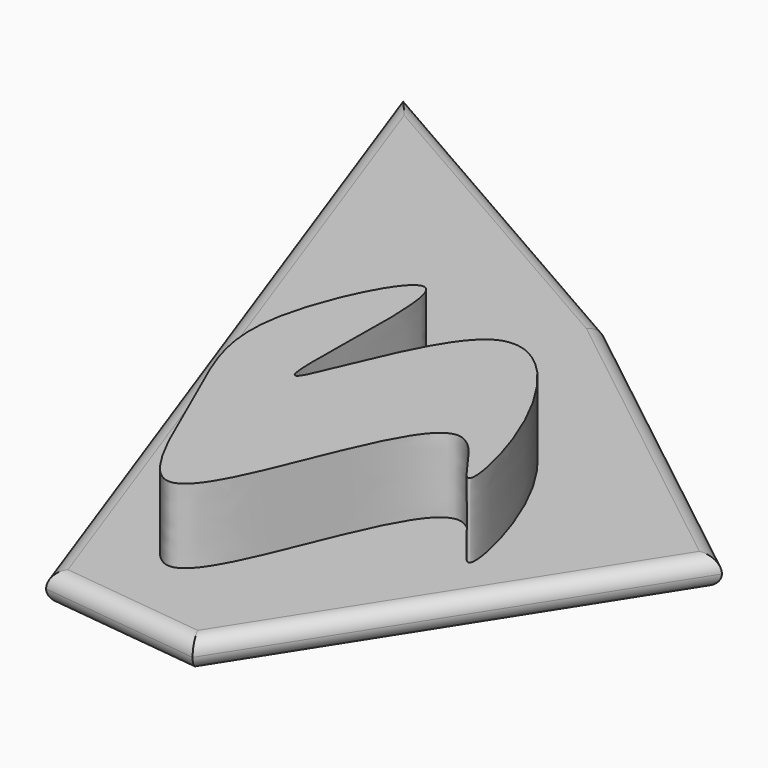
from build123d import *

# Parameters (mm, degrees)
F1_DEPTH    = 10
F2_R        = 5.08
F3_T1_DEPTH = 80.9842186748
F3_T3_DEPTH = 174.5076181059
F3_T5_DEPTH = 187.7665216843
F3_T7_DEPTH = 197.3953695309
F3_T9_DEPTH = 319.5650724593
F5_DEPTH    = 25.4


# Not quite as in the source:
# - a fillet or chamfer that OpenCascade refuses, or shapes differently, is made with other operations: its cross-section is extruded or revolved along the edge and cut away or added


with BuildPart() as f1:
    # F0 (on Top) → F1 (new body)
    with BuildSketch(Plane.XY):
        Polygon((96.3573604822, 27.2471159697), (-11.3680064678, 111.8755862117), (-138.5813802481, 184.7751736641), (-38.9760136604, -92.0266956091), (16.2400007248, -98.5227078199), align=None)
    extrude(amount=F1_DEPTH)

    # F2
    f2_edges = [f1.edges().sort_by_distance(p)[0] for p in [
        (-11.368006, -95.274702, 10),
        (56.298681, -35.637796, 10),
        (42.494677, 69.561351, 10),
        (-74.974693, 148.32538, 10),
        (-88.778697, 46.374239, 10),
    ]]
    fillet(f2_edges, radius=F2_R)

    # F3: fillet of radius 5.08 on 5 edges, made by hand

    # F3_s2 → F3_t1 (cut)
    with BuildSketch(Plane(origin=(-40.3717884669, 4.7496298633, 0), x_dir=(0, 0, 1), z_dir=(0.9931505824, -0.1168414342, 0))):
        with BuildLine():
            ThreePointArc((4.92, 95.9503796722), (1.4317675513, 94.4079813111), (0, 90.8728999824))
            Line((0, 90.8728999824), (-0.1016, 90.8728999824))
            Line((-0.1016, 90.8728999824), (-0.1016, 95.9503796722))
            Line((-0.1016, 95.9503796722), (0, 96.0519796722))
            ThreePointArc((0, 96.0519796722), (2.46, 96.0519796722), (4.9168, 96.051929266))
            Line((4.9168, 96.051929266), (4.92, 95.9503796722))
        make_face()
    extrude(amount=F3_T1_DEPTH, mode=Mode.SUBTRACT)

    # F3_s4 → F3_t3 (cut)
    with BuildSketch(Plane(origin=(-46.7764695351, -73.4306316227, 0), x_dir=(0, 0, 1), z_dir=(0.5372669108, 0.8434122755, 0))):
        with BuildLine():
            ThreePointArc((0, 61.5525271533), (1.4317675513, 65.0876084819), (4.92, 66.630006843))
            Line((4.92, 66.630006843), (4.9168, 66.7315564368))
            ThreePointArc((4.9168, 66.7315564368), (2.46, 66.731606843), (0, 66.731606843))
            Line((0, 66.731606843), (-0.1016, 66.630006843))
            Line((-0.1016, 66.630006843), (-0.1016, 61.5525271533))
            Line((-0.1016, 61.5525271533), (0, 61.5525271533))
        make_face()
    extrude(amount=F3_T3_DEPTH, mode=Mode.SUBTRACT)

    # F3_s6 → F3_t5 (cut)
    with BuildSketch(Plane(origin=(56.3299245333, -44.2524864577, 0), x_dir=(0, 0, 1), z_dir=(-0.7863640458, 0.6177633749, 0))):
        with BuildLine():
            ThreePointArc((0, 75.8747208727), (1.4317675513, 79.4098022013), (4.92, 80.9522005625))
            Line((4.92, 80.9522005625), (4.9168, 81.0537501563))
            ThreePointArc((4.9168, 81.0537501563), (2.46, 81.0538005625), (0, 81.0538005625))
            Line((0, 81.0538005625), (-0.1016, 80.9522005625))
            Line((-0.1016, 80.9522005625), (-0.1016, 75.8747208727))
            Line((-0.1016, 75.8747208727), (0, 75.8747208727))
        make_face()
    extrude(amount=F3_T5_DEPTH, mode=Mode.SUBTRACT)

    # F3_s8 → F3_t7 (cut)
    with BuildSketch(Plane(origin=(-23.7789855791, 13.6265408836, 0), x_dir=(0, 0, 1), z_dir=(-0.8676365908, 0.4971989001, 0))):
        with BuildLine():
            ThreePointArc((0, 86.3377122117), (1.4317675513, 89.8727935404), (4.92, 91.4151919015))
            Line((4.92, 91.4151919015), (4.9168, 91.5167414953))
            ThreePointArc((4.9168, 91.5167414953), (2.46, 91.5167919015), (0, 91.5167919015))
            Line((0, 91.5167919015), (-0.1016, 91.4151919015))
            Line((-0.1016, 91.4151919015), (-0.1016, 86.3377122117))
            Line((-0.1016, 86.3377122117), (0, 86.3377122117))
        make_face()
    extrude(amount=F3_T7_DEPTH, mode=Mode.SUBTRACT)

    # F3_s10 → F3_t9 (cut)
    with BuildSketch(Plane(origin=(-79.0528289065, 219.6866651096, 0), x_dir=(0, 0, 1), z_dir=(0.3385891432, -0.9409343187, 0))):
        with BuildLine():
            ThreePointArc((4.92, 67.8331088759), (1.4317675513, 66.2907105148), (0, 62.7556291862))
            Line((0, 62.7556291862), (-0.1016, 62.7556291862))
            Line((-0.1016, 62.7556291862), (-0.1016, 67.8331088759))
            Line((-0.1016, 67.8331088759), (0, 67.9347088759))
            ThreePointArc((0, 67.9347088759), (2.46, 67.9347088759), (4.9168, 67.9346584697))
            Line((4.9168, 67.9346584697), (4.92, 67.8331088759))
        make_face()
    extrude(amount=F3_T9_DEPTH, mode=Mode.SUBTRACT)

    # F4 (on face) → F5 (join)
    with BuildSketch(Plane.XY.offset(10)):
        with BuildLine():
            add(Edge.make_bspline(
                [(-31.2644466758, 60.5830699205), (-36.0298589944, 66.4844032809), (-62.2139736916, 15.5009480269), (-42.2468798531, -19.940148882), (-18.8038565995, -82.4170143142), (1.9832701602, -49.3566571297), (24.7156161179, 21.5969310396), (51.1884621444, -34.1149723312), (40.5368400052, 21.0125630517), (-3.4050375117, 78.1301949532), (-36.095899728, -46.0942022167), (-25.5245888635, 53.4750145988), (-31.2644466758, 60.5830699205)],
                knots=[0, 0, 0, 0, 0.0974879994, 0.205191583, 0.3109290902, 0.3885576148, 0.5016216887, 0.5752621146, 0.664965491, 0.7698997389, 0.8825773684, 1, 1, 1, 1], degree=3))
        make_face()
    extrude(amount=F5_DEPTH)


solid = f1.part
